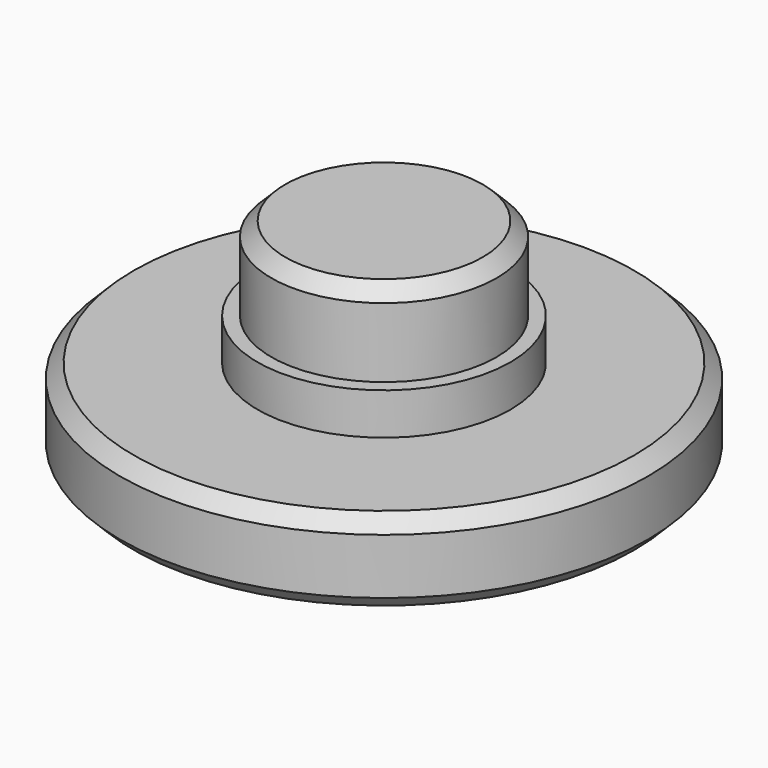
from build123d import *

# Parameters (mm, degrees)
F0_R         = 9.5
F1_DEPTH     = 3
F2_R         = 4.05
F3_DEPTH     = 4.5
F4_SIZE      = 0.5
F5_R         = 4.55
F6_DEPTH     = 1.5
F7_TEXT_SIZE = 13.8888888889
F8_DEPTH     = 1


# Not quite as in the source:
# - Text() gives the source's letters only with a copy of the font that has no kerning and outlines rounded to 1/6400 em; it was checked with that copy


with BuildPart() as f1:
    # F0 (on Top) → F1 (new body)
    with BuildSketch(Plane.XY):
        Circle(F0_R)
    extrude(amount=F1_DEPTH)

    # F2 (on face) → F3 (join)
    with BuildSketch(Plane.XY.offset(3)):
        Circle(F2_R)
    extrude(amount=F3_DEPTH)

    # F4
    f4_edges = [f1.edges().sort_by_distance(p)[0] for p in [
        (-4.05, 0, 7.5),
        (-9.5, 0, 3),
        (-9.5, 0, 0),
    ]]
    chamfer(f4_edges, length=F4_SIZE)

    # F5 (on face) → F6 (join)
    with BuildSketch(Plane.XY.offset(3)):
        Circle(F5_R)
    extrude(amount=F6_DEPTH)

    # F7 (on face) → F8 (cut)
    with BuildSketch(Plane(origin=(0, 0, 0), x_dir=(1, 0, 0), z_dir=(0, 0, -1))):
        with Locations((-4.5106336806, -5)):
            Text('L', F7_TEXT_SIZE, font='Arimo', font_style=FontStyle.BOLD, text_align=(TextAlign.LEFT, TextAlign.BOTTOM))
    extrude(amount=-F8_DEPTH, mode=Mode.SUBTRACT)


solid = f1.part
